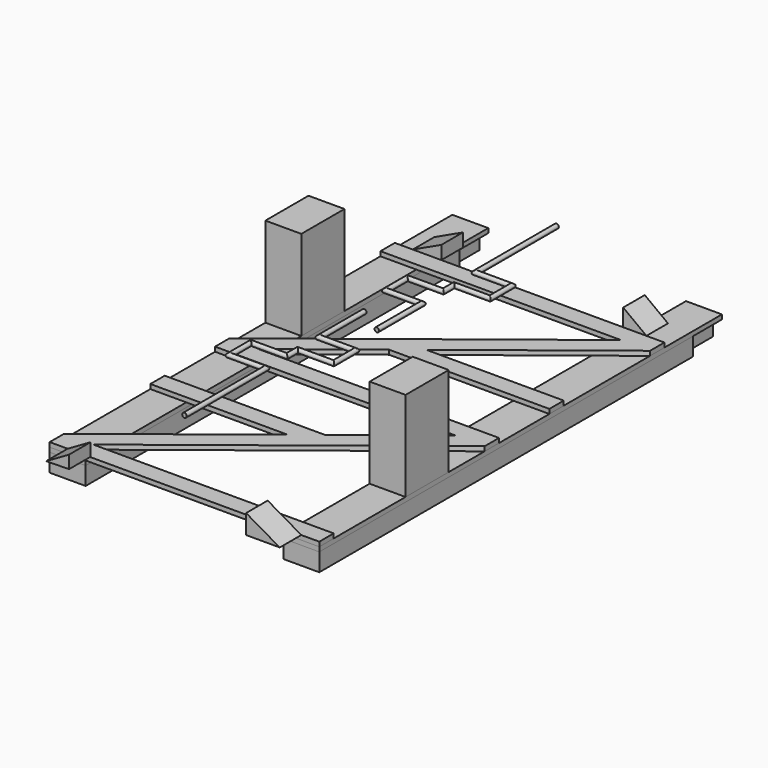
from build123d import *

# Parameters (mm, degrees)
F2_START  = -25.4
F1_W      = 203.2
F1_H      = 304.8
F1_H_2    = 1524
F2_DEPTH  = 101.6
F1_H_3    = 609.6
F3_DEPTH  = 508
F4_DEPTH  = 508
F1_W_2    = 50.8
F1_H_4    = 203.2
F6_DEPTH  = 25.4
F7_W      = 558.8
F7_H      = 101.6
F7_W_2    = 203.2
F8_DEPTH  = 25.4
F11_R     = 12.7
F13_R     = 12.7
F15_DEPTH = 152.4
F16_DEPTH = 152.4


with BuildPart() as f2:
    # F1 (on Top) → F2 (new body)
    with BuildSketch(Plane.XY.offset(F2_START)):
        Polygon((-762, 1422.4), (-762, 1219.2), (-660.4, 1219.2), (-660.4, 1422.4), (-711.2, 1422.4), align=None)
        Polygon((-660.4, 1219.2), (-762, 1219.2), (-762, 609.6), (-558.8, 609.6), (-558.8, 1219.2), align=None)
        Polygon((-660.4, 1422.4), (-660.4, 1219.2), (-558.8, 1219.2), (-558.8, 1422.4), (-609.6, 1422.4), align=None)
        with Locations((-660.4, 457.2)):
            Rectangle(F1_W, F1_H)
        Polygon((-711.2, 1422.4), (-660.4, 1422.4), (-609.6, 1422.4), (-609.6, 1625.6), (-711.2, 1625.6), align=None)
        with Locations((-660.4, -457.2)):
            Rectangle(F1_W, F1_H_2)
        Polygon((-660.4, 1651), (-711.2, 1625.6), (-609.6, 1625.6), align=None)
    extrude(amount=-F2_DEPTH)


with BuildPart() as f2b:
    # F1 (on Top) → F2, piece 2 (new body)
    with BuildSketch(Plane.XY.offset(F2_START)):
        Polygon((660.4, 1219.2), (558.8, 1219.2), (558.8, -304.8), (762, -304.8), (762, 1219.2), align=None)
        Polygon((558.8, 1422.4), (558.8, 1219.2), (660.4, 1219.2), (660.4, 1422.4), (609.6, 1422.4), align=None)
        with Locations((660.4, -457.2)):
            Rectangle(F1_W, F1_H)
        Polygon((660.4, 1422.4), (660.4, 1219.2), (762, 1219.2), (762, 1422.4), (711.2, 1422.4), align=None)
        with Locations((660.4, -914.4)):
            Rectangle(F1_W, F1_H_3)
        Polygon((609.6, 1422.4), (660.4, 1422.4), (711.2, 1422.4), (711.2, 1625.6), (609.6, 1625.6), align=None)
    extrude(amount=-F2_DEPTH)


with BuildPart() as f3:
    # F1 (on Top) → F3 (new body)
    with BuildSketch(Plane.XY):
        with Locations((-660.4, 457.2)):
            Rectangle(F1_W, F1_H)
    extrude(amount=F3_DEPTH)


with BuildPart() as f4:
    # F1 (on Top) → F4 (new body)
    with BuildSketch(Plane.XY):
        with Locations((660.4, -457.2)):
            Rectangle(F1_W, F1_H)
    extrude(amount=F4_DEPTH)


with BuildPart() as f6:
    # F1 (on Top) → F6 (new body)
    with BuildSketch(Plane.XY):
        with Locations((-736.6, 1524)):
            Rectangle(F1_W_2, F1_H_4)
        Polygon((-711.2, 1422.4), (-660.4, 1422.4), (-609.6, 1422.4), (-609.6, 1625.6), (-711.2, 1625.6), align=None)
        with Locations((-584.2, 1524)):
            Rectangle(F1_W_2, F1_H_4)
        Polygon((-660.4, 1422.4), (-660.4, 1219.2), (-558.8, 1219.2), (-558.8, 1422.4), (-609.6, 1422.4), align=None)
        Polygon((-762, 1422.4), (-762, 1219.2), (-660.4, 1219.2), (-660.4, 1422.4), (-711.2, 1422.4), align=None)
        Polygon((-660.4, 1219.2), (-762, 1219.2), (-762, 609.6), (-558.8, 609.6), (-558.8, 1219.2), align=None)
        with Locations((-660.4, -457.2)):
            Rectangle(F1_W, F1_H_2)
        with Locations((-660.4, 457.2)):
            Rectangle(F1_W, F1_H)
    extrude(amount=-F6_DEPTH)


with BuildPart() as f6b:
    # F1 (on Top) → F6, piece 2 (new body)
    with BuildSketch(Plane.XY):
        Polygon((660.4, 1219.2), (558.8, 1219.2), (558.8, -304.8), (762, -304.8), (762, 1219.2), align=None)
        with Locations((660.4, -914.4)):
            Rectangle(F1_W, F1_H_3)
        with Locations((584.2, 1524)):
            Rectangle(F1_W_2, F1_H_4)
        Polygon((609.6, 1422.4), (660.4, 1422.4), (711.2, 1422.4), (711.2, 1625.6), (609.6, 1625.6), align=None)
        with Locations((736.6, 1524)):
            Rectangle(F1_W_2, F1_H_4)
        Polygon((660.4, 1422.4), (660.4, 1219.2), (762, 1219.2), (762, 1422.4), (711.2, 1422.4), align=None)
        Polygon((558.8, 1422.4), (558.8, 1219.2), (660.4, 1219.2), (660.4, 1422.4), (609.6, 1422.4), align=None)
        with Locations((660.4, -457.2)):
            Rectangle(F1_W, F1_H)
    extrude(amount=-F6_DEPTH)


with BuildPart() as f8:
    # F7 (on Top) → F8 (new body)
    with BuildSketch(Plane.XY):
        Polygon((0, 648.7744153468), (-558.8, 210.2598440925), (-558.8, 81.111013399), (-144.2835902197, 406.4), (-14.8145059026, 508), (0, 519.6255846532), align=None)
        Polygon((-558.8, 210.2598440925), (-762, 50.8), (-597.4253853296, 50.8), (-558.8, 81.111013399), align=None)
        Polygon((558.8, 1087.288986601), (0, 648.7744153468), (0, 519.6255846532), (558.8, 958.1401559075), align=None)
        Polygon((597.4253853296, 1117.6), (558.8, 1087.288986601), (558.8, 958.1401559075), (762, 1117.6), align=None)
        Polygon((762, 1219.2), (558.8, 1219.2), (558.8, 1117.6), (597.4253853296, 1117.6), (762, 1117.6), align=None)
        with Locations((279.4, 1168.4)):
            Rectangle(F7_W, F7_H)
        with Locations((-279.4, 1168.4)):
            Rectangle(F7_W, F7_H)
        with Locations((-660.4, 1168.4)):
            Rectangle(F7_W_2, F7_H)
        with Locations((-279.4, 0)):
            Rectangle(F7_W, F7_H)
        Polygon((-597.4253853296, 50.8), (-762, 50.8), (-762, -50.8), (-558.8, -50.8), (-558.8, 50.8), align=None)
        with Locations((279.4, 0)):
            Rectangle(F7_W, F7_H)
        Polygon((558.8, 50.8), (558.8, -50.8), (597.4253853296, -50.8), (762, -50.8), (762, 50.8), align=None)
        Polygon((558.8, -81.111013399), (144.2835902197, -406.4), (14.8145059026, -508), (0, -519.6255846533), (0, -648.7744153467), (558.8, -210.2598440925), align=None)
        Polygon((597.4253853296, -50.8), (558.8, -81.111013399), (558.8, -210.2598440925), (762, -50.8), align=None)
        Polygon((0, -519.6255846533), (-558.8, -958.1401559075), (-558.8, -1087.288986601), (0, -648.7744153467), align=None)
        Polygon((-558.8, -958.1401559075), (-762, -1117.6), (-597.4253853296, -1117.6), (-558.8, -1087.288986601), align=None)
        with Locations((-279.4, -1168.4)):
            Rectangle(F7_W, F7_H)
        Polygon((-597.4253853296, -1117.6), (-762, -1117.6), (-762, -1219.2), (-558.8, -1219.2), (-558.8, -1117.6), align=None)
        with Locations((279.4, -1168.4)):
            Rectangle(F7_W, F7_H)
        with Locations((660.4, -1168.4)):
            Rectangle(F7_W_2, F7_H)
        with Locations((-279.4, -457.2)):
            Rectangle(F7_W, F7_H)
        with Locations((-660.4, -457.2)):
            Rectangle(F7_W_2, F7_H)
        Polygon((144.2835902197, -406.4), (0, -406.4), (0, -508), (14.8145059026, -508), align=None)
        Polygon((-14.8145059026, 508), (-144.2835902197, 406.4), (0, 406.4), (0, 508), align=None)
        with Locations((660.4, 457.2)):
            Rectangle(F7_W_2, F7_H)
        with Locations((279.4, 457.2)):
            Rectangle(F7_W, F7_H)
    extrude(amount=F8_DEPTH)


with BuildPart() as f12:
    # F12: sweep along a path in F5
    with BuildLine(Plane.XY.offset(406.4)) as f12_path:
        Line((152.4, 1219.2), (152.4, 647.7))
        Line((152.4, 647.7), (355.6, 647.7))
        Line((355.6, 647.7), (355.6, 495.3))
        Line((355.6, 495.3), (152.4, 495.3))
        Line((152.4, 495.3), (152.4, 419.1))
        Line((152.4, 419.1), (-50.8, 419.1))
        Line((-50.8, 419.1), (-50.8, 266.7))
        Line((-50.8, 266.7), (152.4, 266.7))
        Line((152.4, 266.7), (152.4, -50.8))
    # F11 (on offset) → F12 (sweep)
    with BuildSketch(Plane(origin=(0, 1219.2, 0), x_dir=(-1, 0, 0), z_dir=(0, 1, 0))):
        with Locations((-152.4, 406.4)):
            Circle(F11_R)
    sweep(path=f12_path.line, transition=Transition.RIGHT)


with BuildPart() as f14:
    # F14: sweep along a path in F5
    with BuildLine(Plane.XY.offset(406.4)) as f14_path:
        Line((0, -1219.2), (0, -647.7))
        Line((0, -647.7), (-203.2, -647.7))
        Line((-203.2, -647.7), (-203.2, -495.3))
        Line((-203.2, -495.3), (0, -495.3))
        Line((0, -495.3), (0, -419.1))
        Line((0, -419.1), (203.2, -419.1))
        Line((203.2, -419.1), (203.2, -266.7))
        Line((203.2, -266.7), (0, -266.7))
        Line((0, -266.7), (0, 50.8))
    # F13 (on offset) → F14 (sweep)
    with BuildSketch(Plane.XZ.offset(1219.2)):
        with Locations((0, 406.4)):
            Circle(F13_R)
    sweep(path=f14_path.line, transition=Transition.RIGHT)


with BuildPart() as f15:
    # F13 (on offset) → F15 (new body)
    with BuildSketch(Plane.XZ.offset(1219.2)):
        Polygon((-530.3294147081, 27.9253141867), (-530.3294147081, 100.4407222838), (-660.4, 25.4), align=None)
    extrude(amount=F15_DEPTH)


with BuildPart() as f15b:
    # F13 (on offset) → F15, piece 2 (new body)
    with BuildSketch(Plane.XZ.offset(1219.2)):
        Polygon((660.4, 25.4), (470.2320303052, 135.1122902086), (470.2320303052, 25.4), align=None)
    extrude(amount=F15_DEPTH)


with BuildPart() as f16:
    # F11 (on offset) → F16 (new body)
    with BuildSketch(Plane(origin=(0, 1219.2, 0), x_dir=(-1, 0, 0), z_dir=(0, 1, 0))):
        Polygon((-529.2000174522, 123.7999869108), (-660.4, 25.4), (-529.2000174522, 25.4), align=None)
    extrude(amount=F16_DEPTH)


with BuildPart() as f16b:
    # F11 (on offset) → F16, piece 2 (new body)
    with BuildSketch(Plane(origin=(0, 1219.2, 0), x_dir=(-1, 0, 0), z_dir=(0, 1, 0))):
        Polygon((498.9599585533, 25.4), (660.4, 25.4), (498.9599585533, 101.0750194281), align=None)
    extrude(amount=F16_DEPTH)


solid = Compound([f2.part, f2b.part, f3.part, f4.part, f6.part, f6b.part, f8.part, f12.part, f14.part, f15.part, f15b.part, f16.part, f16b.part])
